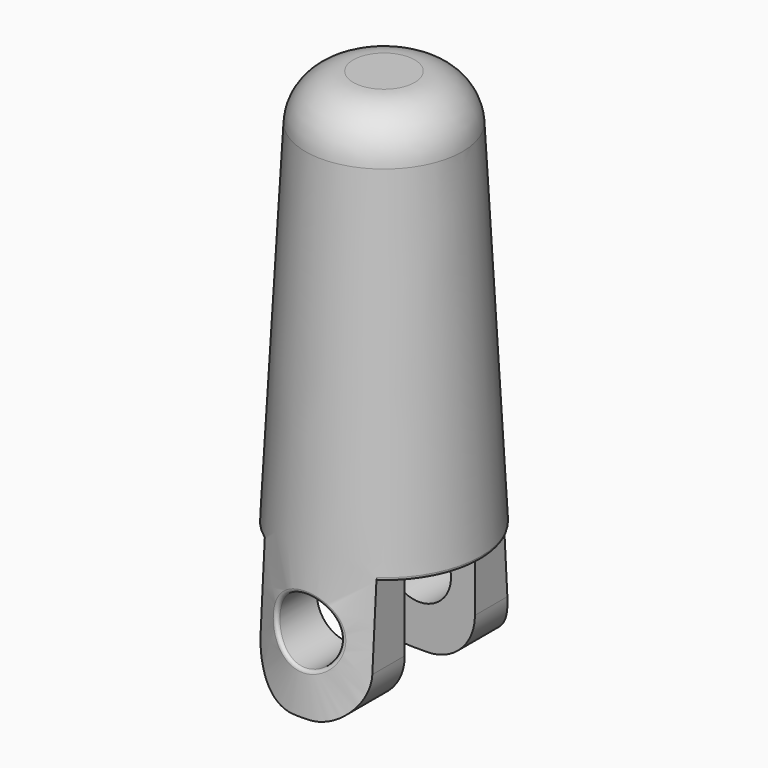
from build123d import *

# Parameters (mm, degrees)
F0_R          = 6.5
F1_DEPTH      = 33
F1_TAPER      = 3
F2_R          = 3
F3_W          = 1.5
F3_H          = 5.5
F3_W_2        = 7
F4_DEPTH      = 8
F5_R          = 2
F6_DEPTH      = 25
F6_DEPTH_BACK = 25
F7_T          = 1
F8_R          = 0.2
F9_R          = 3


# Not quite as in the source:
# - a shell that OpenCascade refuses in one call is made with other operations: the cavity is built on its own and cut out


with BuildPart() as f1:
    # F0 (on Top) → F1 (new body)
    with BuildSketch(Plane.XY):
        Circle(F0_R)
    extrude(amount=F1_DEPTH, taper=F1_TAPER)

    # F2
    f2_edges = [f1.edges().sort_by_distance(p)[0] for p in [
        (-4.770543, 0, 33),
    ]]
    fillet(f2_edges, radius=F2_R)

    # F3 (on Top) → F4 (cut)
    with BuildSketch(Plane.XY):
        Polygon((5, 2.75), (5, -2.75), (3.5, -2.75), (3.5, -6.25), (6.5, -6.25), (6.5, 6.25), (3.5, 6.25), (3.5, 2.75), align=None)
        with Locations((4.25, 0)):
            Rectangle(F3_W, F3_H)
        Rectangle(F3_W_2, F3_H)
        Polygon((-3.5, -6.25), (-3.5, -2.75), (-5, -2.75), (-5, 2.75), (-3.5, 2.75), (-3.5, 6.25), (-6.5, 6.25), (-6.5, -6.25), align=None)
        with Locations((-4.25, 0)):
            Rectangle(F3_W, F3_H)
    extrude(amount=F4_DEPTH, mode=Mode.SUBTRACT)

    # F5 (on face) → F6 (cut, two sides)
    with BuildSketch(Plane(origin=(0, -2.75, 0), x_dir=(-1, 0, 0), z_dir=(0, 1, 0))) as f6_sk:
        with Locations((0, 4.5984359458)):
            Circle(F5_R)
    extrude(amount=F6_DEPTH, mode=Mode.SUBTRACT)
    extrude(f6_sk.sketch, amount=-F6_DEPTH_BACK, mode=Mode.SUBTRACT)

    # F7: shell of thickness 1, made by hand


with BuildPart() as f7_core1:
    # F7_t2: copy of F1
    add(f1.part)

    # the walls: a layer under each face that stays
    f7_faces = [f7_core1.faces().sort_by_distance(p)[0] for p in [
        (-5.7097690939, 0, 15.0785039344),
        (3.5, -4.1136127875, 4),
        (0, -4.625, 0),
        (-3.5, -4.1136127875, 4),
        (-3.5, 4.1136127875, 4),
        (0, 4.625, 0),
        (3.5, 4.1136127875, 4),
        (-3.9887133106, 0, 32.176123113),
        (2, 4.5569343282, 4.5984359458),
        (2, -4.5569343282, 4.5984359458),
        (-2.3333333333, -2.75, 6.6666666667),
        (2.3333333333, 2.75, 6.6666666667),
        (0, 0, 33),
    ]]
    thicken(f7_faces, amount=-F7_T, mode=Mode.SUBTRACT)


with BuildPart() as f1_1:
    add(f1.part)

    # what is left inside the walls is the cavity
    f7_cavity = [f7_core1.part.solids().sort_by_distance(p)[0] for p in [
        (0, -4.859979, 1.588436),
        (-4.744134, 0, 14.205533),
        (0, 4.859979, 1.588436),
    ]]
    add(f7_cavity, mode=Mode.SUBTRACT)

    # F8
    f8_edges = [f1_1.edges().sort_by_distance(p)[0] for p in [
        (1.999873, -5.932154, 4.575894),
        (5.397127, -2.801142, 8),
        (-6.080738, 0, 8),
        (5.397127, 2.801142, 8),
        (1.999882, 5.932105, 4.576739),
    ]]
    fillet(f8_edges, radius=F8_R)

    # F9
    f9_edges = [f1_1.edges().sort_by_distance(p)[0] for p in [
        (3.5, -4.113613, 0),
        (3.5, 4.113613, 0),
        (-3.5, 4.113613, 0),
        (-3.5, -4.113613, 0),
    ]]
    fillet(f9_edges, radius=F9_R)


solid = f1_1.part
